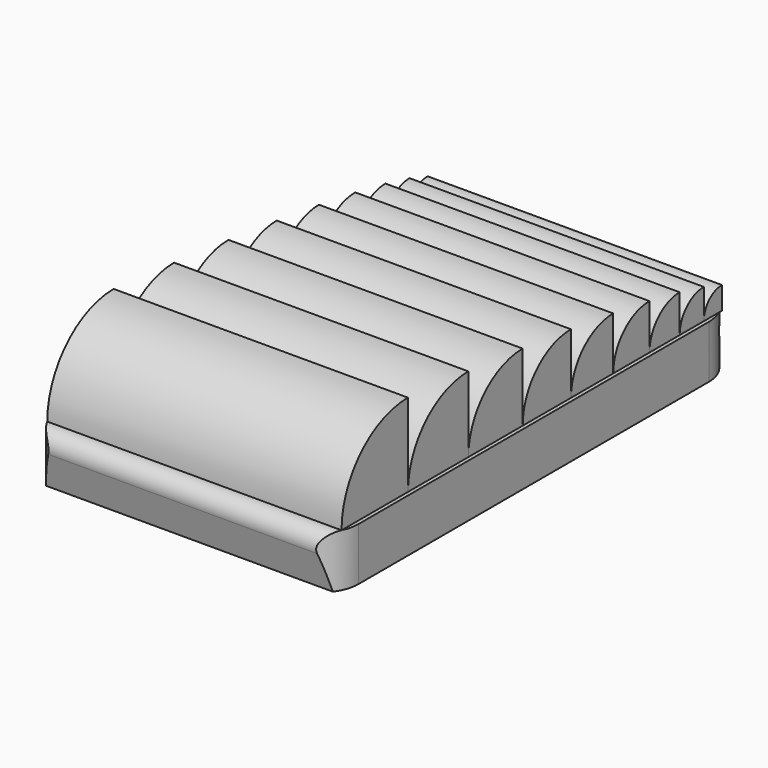
from build123d import *

# Parameters (mm, degrees)
F0_W        = 200
F0_H        = 340
F1_DEPTH    = 35
F2_W        = 15
F2_H        = 130
F3_DEPTH    = 0.5
F4_R        = 25
F5_T1_DEPTH = 357.7701999818
F6_R        = 10
F8_DEPTH    = 97.478


# Not quite as in the source:
# - a fillet or chamfer that OpenCascade refuses, or shapes differently, is made with other operations: its cross-section is extruded or revolved along the edge and cut away or added


with BuildPart() as f1:
    # F0 (on Top) → F1 (new body)
    with BuildSketch(Plane.XY):
        Rectangle(F0_W, F0_H)
    extrude(amount=F1_DEPTH)

    # F2 (on face) → F3 (cut)
    with BuildSketch(Plane(origin=(0, 0, 0), x_dir=(1, 0, 0), z_dir=(0, 0, -1))):
        with Locations((-50, 95)):
            Rectangle(F2_W, F2_H)
        with Locations((50, 95)):
            Rectangle(F2_W, F2_H)
        with Locations((-50, -95)):
            Rectangle(F2_W, F2_H)
        with Locations((50, -95)):
            Rectangle(F2_W, F2_H)
    extrude(amount=-F3_DEPTH, mode=Mode.SUBTRACT)

    # F4
    f4_edges = [f1.edges().sort_by_distance(p)[0] for p in [
        (100, -170, 17.5),
        (-100, -170, 17.5),
        (100, 170, 17.5),
        (-100, 170, 17.5),
    ]]
    fillet(f4_edges, radius=F4_R)

    # F5: chamfer of 40 x 10 on 2 edges, made by hand

    # F5_s2 → F5_t1 (cut)
    with BuildSketch(Plane.YZ.offset(-178.8850999909)):
        Polygon((-160, 0), (-170, 40), (-170, 0), align=None)
        Polygon((170, 40), (160, 0), (170, 0), align=None)
    extrude(amount=F5_T1_DEPTH, mode=Mode.SUBTRACT)

    # F6
    f6_edges = [f1.edges().sort_by_distance(p)[0] for p in [
        (0, -168.75, 35),
    ]]
    fillet(f6_edges, radius=F6_R)

    # F7 (on Right) → F8 (join, symmetric)
    with BuildSketch(Plane.YZ):
        with BuildLine():
            Line((-155.942235936, 35), (-100.942235936, 35))
            Line((-100.942235936, 35), (-100.942235936, 90))
            ThreePointArc((-100.942235936, 90), (-139.8331089012, 73.8908729653), (-155.942235936, 35))
        make_face()
        with BuildLine():
            ThreePointArc((-50.942235936, 85), (-86.2975749953, 70.3553390593), (-100.942235936, 35))
            Line((-100.942235936, 35), (-50.942235936, 35))
            Line((-50.942235936, 35), (-50.942235936, 85))
        make_face()
        with BuildLine():
            ThreePointArc((-5.942235936, 80), (-37.7620410894, 66.8198051534), (-50.942235936, 35))
            Line((-50.942235936, 35), (-5.942235936, 35))
            Line((-5.942235936, 35), (-5.942235936, 75))
            Line((-5.942235936, 75), (-5.942235936, 80))
        make_face()
        with BuildLine():
            ThreePointArc((159.057764064, 50), (148.4511623462, 45.6066017178), (144.057764064, 35))
            Line((144.057764064, 35), (159.057764064, 35))
            Line((159.057764064, 35), (159.057764064, 50))
        make_face()
        with BuildLine():
            ThreePointArc((34.057764064, 75), (5.7734928166, 63.2842712475), (-5.942235936, 35))
            Line((-5.942235936, 35), (34.057764064, 35))
            Line((34.057764064, 35), (34.057764064, 70))
            Line((34.057764064, 70), (34.057764064, 75))
        make_face()
        with BuildLine():
            ThreePointArc((69.057764064, 70), (44.3090267225, 59.7487373415), (34.057764064, 35))
            Line((34.057764064, 35), (69.057764064, 35))
            Line((69.057764064, 35), (69.057764064, 65))
            Line((69.057764064, 65), (69.057764064, 70))
        make_face()
        with BuildLine():
            ThreePointArc((99.057764064, 65), (77.8445606284, 56.2132034356), (69.057764064, 35))
            Line((69.057764064, 35), (99.057764064, 35))
            Line((99.057764064, 35), (99.057764064, 60))
            Line((99.057764064, 60), (99.057764064, 65))
        make_face()
        with BuildLine():
            ThreePointArc((124.057764064, 60), (106.3800945344, 52.6776695297), (99.057764064, 35))
            Line((99.057764064, 35), (124.057764064, 35))
            Line((124.057764064, 35), (124.057764064, 55))
            Line((124.057764064, 55), (124.057764064, 60))
        make_face()
        with BuildLine():
            ThreePointArc((144.057764064, 55), (129.9156284403, 49.1421356237), (124.057764064, 35))
            Line((124.057764064, 35), (144.057764064, 35))
            Line((144.057764064, 35), (144.057764064, 50))
            Line((144.057764064, 50), (144.057764064, 55))
        make_face()
    extrude(amount=F8_DEPTH, both=True)


solid = f1.part
